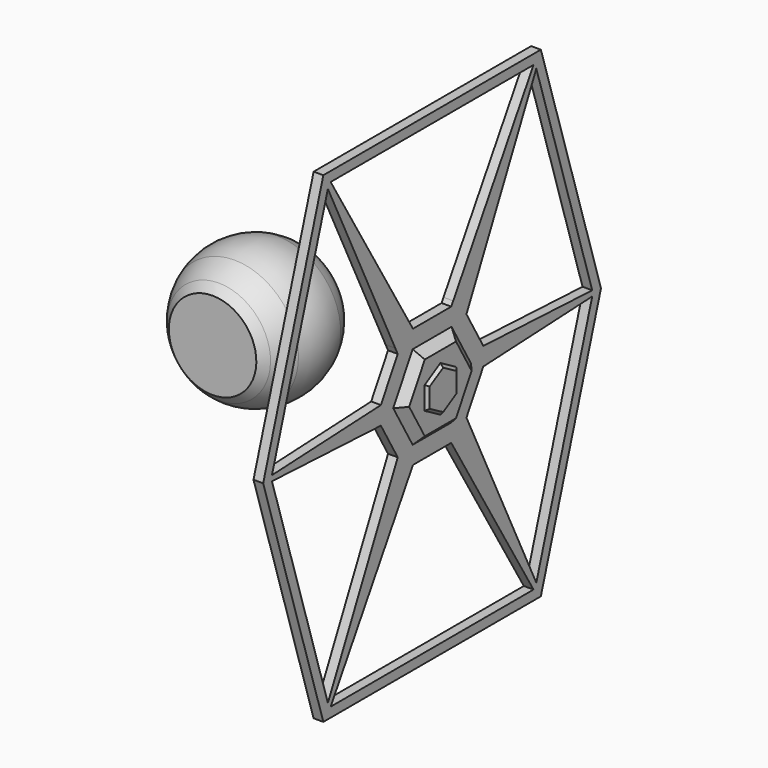
from build123d import *

# Parameters (mm, degrees)
F2_START = 60.25
F2_DEPTH = 3.5
F4_DEPTH = 3.5
F6_DEPTH = 3
F7_SIZE  = 2.99999
F9_DEPTH = 1
F10_SIZE = 0.99999


# Not quite as in the source:
# - a fillet or chamfer is up to 0.001 mm smaller than in the source, because OpenCascade refuses the exact size
# - a feature names something its author has since deleted; it is built from what else it names


with BuildPart() as f1:
    # F0 (on Right) → F1 (revolve)
    with BuildSketch(Plane.YZ):
        with BuildLine():
            ThreePointArc((-16.6007267077, 18.6926689581), (-18.0475959302, 17.2998347143), (-19.3779955618, 15.795356533))
            Line((-19.3779955618, 15.795356533), (-19.3779955618, 0))
            Line((-19.3779955618, 0), (-7.5747272931, 0))
            Line((-7.5747272931, 0), (-16.6007267077, 18.6926689581))
        make_face()
        with BuildLine():
            ThreePointArc((-9.5239152868, 23.1148228981), (-13.2481353859, 21.2011063107), (-16.6007267077, 18.6926689581))
            Line((-16.6007267077, 18.6926689581), (-7.5747272931, 0))
            Line((-7.5747272931, 0), (-4.3816049583, 0))
            Line((-4.3816049583, 0), (0, 7.2834400177))
            Line((0, 7.2834400177), (-9.5239152868, 23.1148228981))
        make_face()
        with BuildLine():
            ThreePointArc((9.5239152868, 23.1148228981), (0, 25), (-9.5239152868, 23.1148228981))
            Line((-9.5239152868, 23.1148228981), (0, 7.2834400177))
            Line((0, 7.2834400177), (9.5239152868, 23.1148228981))
        make_face()
        with BuildLine():
            ThreePointArc((16.6007267077, 18.6926689581), (13.2481353859, 21.2011063107), (9.5239152868, 23.1148228981))
            Line((9.5239152868, 23.1148228981), (0, 7.2834400177))
            Line((0, 7.2834400177), (4.3816049583, 0))
            Line((4.3816049583, 0), (7.5747272931, 0))
            Line((7.5747272931, 0), (16.6007267077, 18.6926689581))
        make_face()
        with BuildLine():
            ThreePointArc((19.3779955618, 15.795356533), (18.0475959302, 17.2998347143), (16.6007267077, 18.6926689581))
            Line((16.6007267077, 18.6926689581), (7.5747272931, 0))
            Line((7.5747272931, 0), (19.3779955618, 0))
            Line((19.3779955618, 0), (19.3779955618, 15.795356533))
        make_face()
    revolve(axis=Axis((0, 9.6889977809, 0), (0, 1, 0)))


with BuildPart() as f2:
    # F0 (on Right) → F2 (new body)
    with BuildSketch(Plane.YZ.offset(F2_START)):
        Polygon((49.0827742896, 86.8854269893), (0, 86.8854269893), (-49.0827742896, 86.8854269893), (-76.2346684933, 0), (-49.0827742896, -86.8854269893), (0, -86.8854269893), (49.0827742896, -86.8854269893), (76.2346684933, 0), align=None)
        Polygon((-45.7817793022, -83.3854269893), (0, -7.2834400177), (45.7817793022, -83.3854269893), (0, -83.3854269893), align=None, mode=Mode.SUBTRACT)
        with BuildLine():
            Line((-47.0317255702, 81.7146747964), (-16.6007267077, 18.6926689581))
            ThreePointArc((-16.6007267077, 18.6926689581), (-13.2481353859, 21.2011063107), (-9.5239152868, 23.1148228981))
            Line((-9.5239152868, 23.1148228981), (-45.7817793022, 83.3854269893))
            Line((-45.7817793022, 83.3854269893), (0, 83.3854269893))
            Line((0, 83.3854269893), (45.7817793022, 83.3854269893))
            Line((45.7817793022, 83.3854269893), (9.5239152868, 23.1148228981))
            ThreePointArc((9.5239152868, 23.1148228981), (13.2481353859, 21.2011063107), (16.6007267077, 18.6926689581))
            Line((16.6007267077, 18.6926689581), (47.0317255702, 81.7146747964))
            Line((47.0317255702, 81.7146747964), (72.5677479141, 0))
            Line((72.5677479141, 0), (47.0317255702, -81.7146747964))
            Line((47.0317255702, -81.7146747964), (7.5747272931, 0))
            Line((7.5747272931, 0), (4.3816049583, 0))
            Line((4.3816049583, 0), (0, -7.2834400177))
            Line((0, -7.2834400177), (-4.3816049583, 0))
            Line((-4.3816049583, 0), (-7.5747272931, 0))
            Line((-7.5747272931, 0), (-47.0317255702, -81.7146747964))
            Line((-47.0317255702, -81.7146747964), (-72.5677479141, 0))
            Line((-72.5677479141, 0), (-47.0317255702, 81.7146747964))
        make_face(mode=Mode.SUBTRACT)
        with BuildLine():
            ThreePointArc((-9.5239152868, 23.1148228981), (-13.2481353859, 21.2011063107), (-16.6007267077, 18.6926689581))
            Line((-16.6007267077, 18.6926689581), (-7.5747272931, 0))
            Line((-7.5747272931, 0), (-4.3816049583, 0))
            Line((-4.3816049583, 0), (0, 7.2834400177))
            Line((0, 7.2834400177), (-9.5239152868, 23.1148228981))
        make_face()
        with BuildLine():
            ThreePointArc((16.6007267077, 18.6926689581), (13.2481353859, 21.2011063107), (9.5239152868, 23.1148228981))
            Line((9.5239152868, 23.1148228981), (0, 7.2834400177))
            Line((0, 7.2834400177), (4.3816049583, 0))
            Line((4.3816049583, 0), (7.5747272931, 0))
            Line((7.5747272931, 0), (16.6007267077, 18.6926689581))
        make_face()
        Polygon((0, 7.2834400177), (-4.3816049583, 0), (0, 0), (4.3816049583, 0), align=None)
        Polygon((0, 0), (-4.3816049583, 0), (0, -7.2834400177), (4.3816049583, 0), align=None)
    extrude(amount=F2_DEPTH)

    # F3 (on face) → F4 (join, through all)
    with BuildSketch(Plane.YZ.offset(63.75)):
        Polygon((23.1128721452, -3.2686013249), (25, 0), (23.1128721452, 3.2686013249), (0, 4.3492764235), (-23.1128721452, 3.2686013249), (-25, 0), (-23.1128721452, -3.2686013249), (0, -4.3492764235), align=None)
        Polygon((12.5, -21.6506350946), (23.1128721452, -3.2686013249), (0, -4.3492764235), (-23.1128721452, -3.2686013249), (-12.5, -21.6506350946), align=None)
        Polygon((0, 4.3492764235), (23.1128721452, 3.2686013249), (12.5, 21.6506350946), (-12.5, 21.6506350946), (-23.1128721452, 3.2686013249), align=None)
        Polygon((-72.2644806371, -0.9704481998), (-23.1128721452, -3.2686013249), (-25, 0), (-23.1128721452, 3.2686013249), (-72.2644806371, 0.9704481998), (-72.5677479141, 0), align=None)
        Polygon((23.1128721452, 3.2686013249), (25, 0), (23.1128721452, -3.2686013249), (72.2644806371, -0.9704481998), (72.5677479141, 0), (72.2644806371, 0.9704481998), align=None)
    extrude(amount=-F4_DEPTH)

    # F5 (on face) → F6 (join)
    with BuildSketch(Plane.YZ.offset(63.75)):
        Polygon((8.7727464607, 15.1948425919), (-8.7727464607, 15.1948425919), (-17.5454929214, 0), (-8.7727464607, -15.1948425919), (8.7727464607, -15.1948425919), (17.5454929214, 0), align=None)
    extrude(amount=F6_DEPTH)

    # F7 (size 3 in the source; OpenCascade refuses exactly that, so slightly less here)
    f7_edges = [f2.edges().sort_by_distance(p)[0] for p in [
        (66.75, -13.15912, 7.597421),
        (66.75, 0, 15.194843),
        (66.75, 13.15912, 7.597421),
        (66.75, 13.15912, -7.597421),
        (66.75, 0, -15.194843),
        (66.75, -13.15912, -7.597421),
    ]]
    chamfer(f7_edges, length=F7_SIZE)

    # F8 (on face) → F9 (join)
    with BuildSketch(Plane.YZ.offset(66.75)):
        Polygon((7.1106306277, -4.105324507), (7.1106306277, 4.105324507), (0, 8.210649014), (-7.1106306277, 4.105324507), (-7.1106306277, -4.105324507), (0, -8.210649014), align=None)
    extrude(amount=F9_DEPTH)

    # F10 (size 1 in the source; OpenCascade refuses exactly that, so slightly less here)
    f10_edges = [f2.edges().sort_by_distance(p)[0] for p in [
        (67.75, -3.555315, 6.157987),
        (67.75, 3.555315, 6.157987),
        (67.75, 7.110631, 0),
        (67.75, 3.555315, -6.157987),
        (67.75, -3.555315, -6.157987),
        (67.75, -7.110631, 0),
    ]]
    chamfer(f10_edges, length=F10_SIZE)


solid = Compound([f1.part, f2.part])
